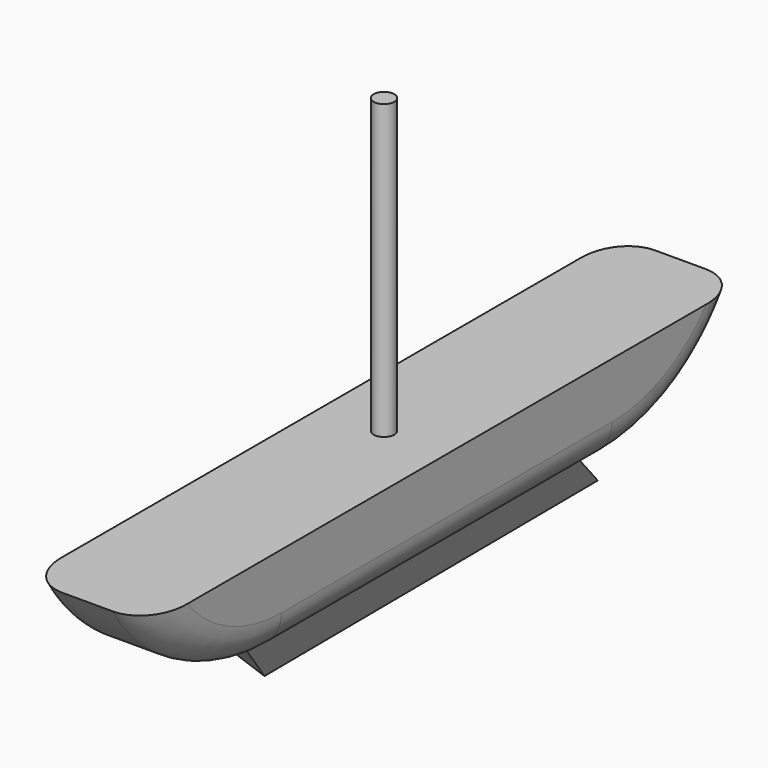
from build123d import *

# Parameters (mm, degrees)
F0_W        = 83.6402177811
F0_H        = 18.8771318644
F1_DEPTH    = 12.7
F2_DEPTH    = 6.35
F3_T4_DEPTH = 183.094881238
F4_T4_DEPTH = 183.094881238
F5_R        = 7.62
F6_R        = 7.62
F7_W        = 2.0920878742
F7_H        = 68.6837211251


# Not quite as in the source:
# - a fillet or chamfer that OpenCascade refuses, or shapes differently, is made with other operations: its cross-section is extruded or revolved along the edge and cut away or added


with BuildPart() as f1:
    # F0 (on Right) → F1 (new body, symmetric)
    with BuildSketch(Plane.YZ):
        with BuildLine():
            ThreePointArc((-74.9276950955, 9.4385659322), (-60.8756748212, -4.3877247968), (-41.8201088905, -9.4385659322))
            Line((-41.8201088905, -9.4385659322), (-74.9276950955, 9.4385659322))
        make_face()
        with BuildLine():
            Line((74.9276950955, 9.4385659322), (41.8201088905, -9.4385659322))
            ThreePointArc((41.8201088905, -9.4385659322), (60.8756748212, -4.3877247968), (74.9276950955, 9.4385659322))
        make_face()
        Polygon((74.9276950955, 9.4385659322), (41.8201088905, 9.4385659322), (41.8201088905, -9.4385659322), align=None)
        Rectangle(F0_W, F0_H)
        Polygon((-41.8201088905, -9.4385659322), (-41.8201088905, 9.4385659322), (-74.9276950955, 9.4385659322), align=None)
    extrude(amount=F1_DEPTH, both=True)

    # F0 (on Right) → F2 (join, symmetric)
    with BuildSketch(Plane.YZ):
        Polygon((41.8201088905, -9.4385659322), (-41.8201088905, -9.4385659322), (-30.2034132183, -21.926516667), (54.0176406503, -21.3456805795), align=None)
    extrude(amount=F2_DEPTH, both=True)

    # F3: chamfer of 19.05 x 6.35 on 1 edges, made by hand


with BuildPart() as f3_tool2:
    # F3_s3 → F3_t4 (new body)
    with BuildSketch(Plane(origin=(0, -79.7879238623, -0.5502627122), x_dir=(1, 0, 0), z_dir=(0, 0.9999762195, 0.0068964024))):
        Polygon((-6.35, 2.6677003539), (0, 21.7177003539), (-6.35, 21.7177003539), align=None)
    extrude(amount=F3_T4_DEPTH)

    split(bisect_by=Plane.XY.offset(-9.4385659322), keep=Keep.BOTTOM)


with BuildPart() as f1_1:
    add(f1.part)

    # F3_t1: cut F3_tool2
    add(f3_tool2.part, mode=Mode.SUBTRACT)

    # F4: chamfer of 6.35 x 19.05 on 1 edges, made by hand


with BuildPart() as f4_tool2:
    # F4_s3 → F4_t4 (new body)
    with BuildSketch(Plane(origin=(0, -79.7879238623, -0.5502627122), x_dir=(1, 0, 0), z_dir=(0, 0.9999762195, 0.0068964024))):
        Polygon((6.35, 2.6677003539), (0, 21.7177003539), (6.35, 21.7177003539), align=None)
    extrude(amount=F4_T4_DEPTH)

    split(bisect_by=Plane.XY.offset(-9.4385659322), keep=Keep.BOTTOM)


with BuildPart() as f1_2:
    add(f1_1.part)

    # F4_t1: cut F4_tool2
    add(f4_tool2.part, mode=Mode.SUBTRACT)

    # F5
    f5_edges = [f1_2.edges().sort_by_distance(p)[0] for p in [
        (-12.7, 60.875675, -4.387725),
        (-12.7, 0, -9.438566),
        (-12.7, -60.875675, -4.387725),
    ]]
    fillet(f5_edges, radius=F5_R)

    # F6
    f6_edges = [f1_2.edges().sort_by_distance(p)[0] for p in [
        (12.7, -60.875675, -4.387725),
        (12.7, 0, -9.438566),
        (12.7, 60.875675, -4.387725),
    ]]
    fillet(f6_edges, radius=F6_R)

    # F7 (on Right) → F8 (revolve)
    with BuildSketch(Plane.YZ):
        with Locations((1.0460439371, 34.3418605626)):
            Rectangle(F7_W, F7_H)
    revolve(axis=Axis((0, 0, 34.3418605626), (0, 0, 1)))


solid = f1_2.part
